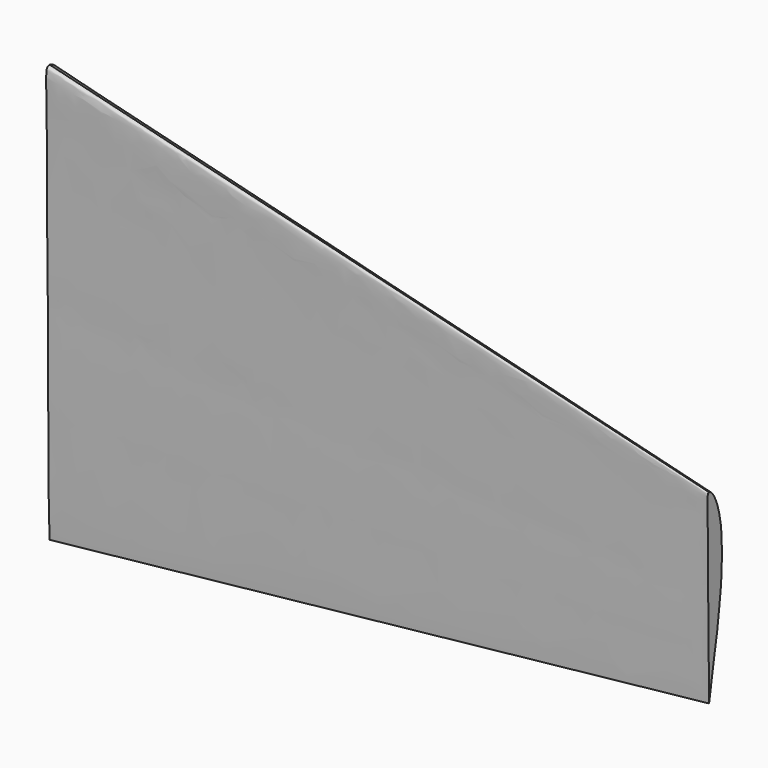
from build123d import *


with BuildPart() as f3:
    # F0 (on Right) → F3 section 0
    with BuildSketch(Plane.YZ):
        with BuildLine():
            add(Edge.make_bspline(
                [(-0.8581783067, 89.0966641903), (-0.0909835006, 88.8375018392), (1.563224164, 88.2787019828), (3.8166245117, 85.6948868237), (7.2769036033, 79.7303238844), (10.3263017721, 71.2559073926), (12.8782546304, 59.6431852965), (14.1220379816, 50.7970965092), (14.5946259905, 40.3812733772), (14.7141619457, 30.792316012), (14.6059947167, 21.4420727085), (14.0276612179, 9.7286883375), (13.2548192102, 0.1374811079), (11.5947174142, -12.4612944717), (10.3935827762, -22.6942842365), (9.1411293748, -32.5543273378), (6.9203884123, -45.066329976), (4.9304517493, -55.8403956919), (3.2204545525, -65.6158467378), (1.8815091078, -75.622213963), (0.3357020939, -84.3559320968), (-0.4706596158, -88.8345114632), (-0.8431484343, -90.9033358097)],
                knots=[0, 0, 0, 0, 0.0259289572, 0.0559074168, 0.0990607278, 0.1498725735, 0.2071251008, 0.2573858131, 0.3107982977, 0.3623398407, 0.4135066245, 0.4700655391, 0.5224390727, 0.581519189, 0.635089011, 0.6874998006, 0.7469121662, 0.8023290394, 0.8546697959, 0.9078000483, 0.9574093727, 1, 1, 1, 1], degree=3))
            add(Edge.make_bspline(
                [(-0.8581783067, 89.0966641903), (-1.404462943, 88.938895504), (-2.4902152414, 88.6253268945), (-2.4171470838, 86.853978738), (-2.8104245698, 85.5401321657), (-2.6480397884, 82.2162290738), (-2.7352274213, 78.3866922604), (-2.594105356, 72.6182494274), (-2.3650949946, 70.0616330556), (-2.4380078188, 65.6685838696), (-2.3999265509, 60.6898081314), (-2.4719402279, 57.0432888195), (-2.1465914902, 49.1284832057), (-2.2526839686, 43.8957450986), (-2.1229527861, 33.8731852803), (-2.0030100309, 21.1298302522), (-2.1584125605, 11.280466173), (-1.6943435842, -0.468552789), (-1.7837254863, -6.1401111108), (-1.7933498326, -18.4803362465), (-1.6230847275, -36.8456317984), (-1.6627691908, -42.0840169933), (-1.2415097852, -57.7937735112), (-1.4530871043, -75.7214856707), (-1.0387131964, -86.0355760548), (-0.8431484343, -90.9033358097)],
                knots=[0, 0, 0, 0, 0.0203275586, 0.0404014537, 0.0599261282, 0.0890506729, 0.1226807844, 0.1617614156, 0.1885435138, 0.2227295591, 0.2593127782, 0.2915111627, 0.3369800906, 0.3754440114, 0.4270931032, 0.4862286015, 0.5393741421, 0.594677489, 0.6336860238, 0.6921988306, 0.7624104014, 0.8010107314, 0.8645716771, 0.9360842774, 1, 1, 1, 1], degree=3))
        make_face()
    # F2 (on offset) → F3 section 1
    with BuildSketch(Plane.YZ.offset(300)):
        with BuildLine():
            add(Edge.make_bspline(
                [(-21.129370218, 32.9211650841), (-20.7883947487, 32.8059818169), (-20.0531913422, 32.5576263252), (-19.0516800765, 31.4092640322), (-17.5137782581, 28.7583471703), (-16.158490183, 24.9919398406), (-15.0242889127, 19.8307300201), (-14.4714963121, 15.8991350036), (-14.261457197, 11.2698802782), (-14.2083301059, 7.0081214492), (-14.2564044299, 2.8524577588), (-14.5134415405, -2.3534908505), (-14.8569268772, -6.6162496192), (-15.5947498977, -12.2157054324), (-16.1285875145, -16.7637008834), (-16.6852334707, -21.1459422618), (-17.6722294541, -26.7068323232), (-18.5566457487, -31.4953059747), (-19.3166445028, -35.839950884), (-19.9117313672, -40.2872252063), (-20.5987567067, -44.1688777102), (-20.9571396887, -46.1593574286), (-21.1226902748, -47.0788349159)],
                knots=[0, 0, 0, 0, 0.0259289572, 0.0559074168, 0.0990607278, 0.1498725735, 0.2071251008, 0.2573858131, 0.3107982977, 0.3623398407, 0.4135066245, 0.4700655391, 0.5224390727, 0.581519189, 0.635089011, 0.6874998006, 0.7469121662, 0.8023290394, 0.8546697959, 0.9078000483, 0.9574093727, 1, 1, 1, 1], degree=3))
            add(Edge.make_bspline(
                [(-21.129370218, 32.9211650841), (-21.3721633897, 32.8510456679), (-21.8547199668, 32.7116818415), (-21.8222452301, 31.9244159942), (-21.9970352238, 31.3404841842), (-21.9248642099, 29.8631939212), (-21.963614269, 28.1611775597), (-21.9008933511, 25.5974251895), (-21.7991109682, 24.4611512464), (-21.8315166679, 22.5086849415), (-21.8145916599, 20.2958957245), (-21.8465977386, 18.6752204748), (-21.7019982996, 15.1575290909), (-21.7491505122, 12.8318677099), (-21.6914922089, 8.3773966796), (-21.6381843177, 2.7136833338), (-21.7072521086, -1.6638118125), (-21.5009992302, -6.8855980178), (-21.5407245201, -9.4062906053), (-21.5450020073, -14.8908351101), (-21.4693286273, -23.0531886887), (-21.4869661665, -25.3813598864), (-21.2997397641, -32.3634738944), (-21.3937741281, -40.3313459653), (-21.2096079468, -44.915386136), (-21.1226902748, -47.0788349159)],
                knots=[0, 0, 0, 0, 0.0203275586, 0.0404014537, 0.0599261282, 0.0890506729, 0.1226807844, 0.1617614156, 0.1885435138, 0.2227295591, 0.2593127782, 0.2915111627, 0.3369800906, 0.3754440114, 0.4270931032, 0.4862286015, 0.5393741421, 0.594677489, 0.6336860238, 0.6921988306, 0.7624104014, 0.8010107314, 0.8645716771, 0.9360842774, 1, 1, 1, 1], degree=3))
        make_face()
    loft()


solid = f3.part
